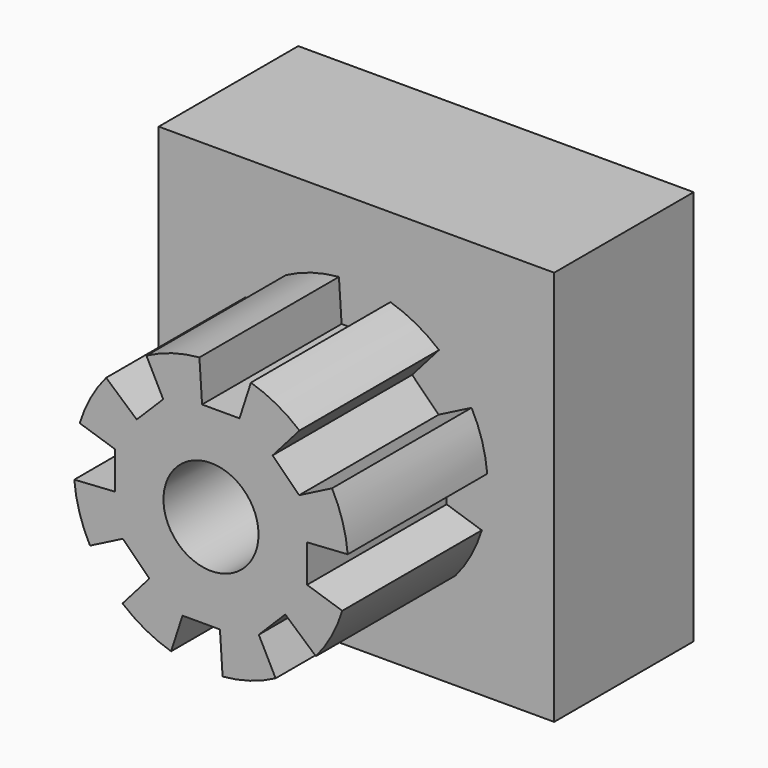
from build123d import *

# Parameters (mm, degrees)
F0_W            = 56.6879622638
F0_H            = 56.6879622638
F1_DEPTH        = 25
F2_R            = 19.6657684011
F3_DEPTH        = 25
F4_R            = 6.8124557353
F5_DEPTH        = 50.001
F7_DEPTH        = 50.001
F7_COPIES_COUNT = 8


# Not quite as in the source:
# - a pattern or mirror of a feature is missing from the dataset's text; its kind, count and spacing are read off the source's solid


with BuildPart() as f1:
    # F0 (on Front) → F1 (new body)
    with BuildSketch(Plane.XZ):
        with Locations((-40.2088612318, 22.6584635675)):
            Rectangle(F0_W, F0_H)
    extrude(amount=F1_DEPTH)


with BuildPart() as f3:
    # F2 (on face) → F3 (new body)
    with BuildSketch(Plane.XZ.offset(25)):
        with Locations((-41.0571657121, 20.8462141454)):
            Circle(F2_R)
    extrude(amount=F3_DEPTH)


with BuildPart() as f5_tool:
    # F4 (on face) → F5 (new body, through all)
    with BuildSketch(Plane.XZ.offset(50)):
        with Locations((-41.0571657121, 20.8462141454)):
            Circle(F4_R)
    extrude(amount=-F5_DEPTH)


with BuildPart() as f1_1:
    add(f1.part)

    # F5: cut by f5_tool
    add(f5_tool.part, mode=Mode.SUBTRACT)


with BuildPart() as f3_1:
    add(f3.part)

    # F5: cut by f5_tool
    add(f5_tool.part, mode=Mode.SUBTRACT)

    # F6 (on face) → F7 (cut, through all)
    with BuildSketch(Plane.XZ.offset(50)):
        Polygon((-19.0042369068, 22.665174678), (-27.28226409, 22.1291541798), (-27.28226409, 16.7617611587), (-19.8002401739, 14.3349375576), align=None)
    f7 = extrude(amount=-F7_DEPTH, mode=Mode.SUBTRACT)

    # F7_copies: F7 ×8 about axis
    f7_copies_axis = Axis((-41.057166, 0, 20.846214), (0, 1, 0))
    for i in range(1, F7_COPIES_COUNT):
        add(f7.rotate(f7_copies_axis, i * 360 / F7_COPIES_COUNT), mode=Mode.SUBTRACT)


solid = Compound([f1_1.part, f3_1.part])
